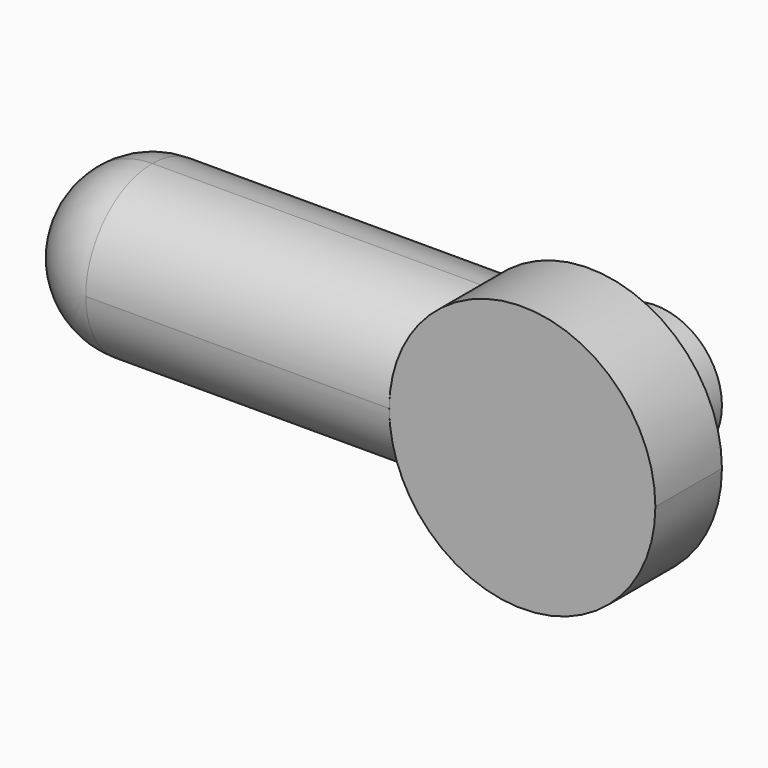
from build123d import *

# Parameters (mm, degrees)
F1_DEPTH = 6.35
F2_R     = 6.3499
F0_R     = 5.08
F3_DEPTH = 6.35
F4_DEPTH = 6.35


# Not quite as in the source:
# - a fillet or chamfer is up to 0.001 mm smaller than in the source, because OpenCascade refuses the exact size


with BuildPart() as f1:
    # F0 (on Front) → F1 (new body, symmetric)
    with BuildSketch(Plane.XZ):
        with BuildLine():
            Line((12.7, 6.35), (-12.7, 6.35))
            Line((-12.7, 6.35), (-12.7, -6.35))
            Line((-12.7, -6.35), (12.7, -6.35))
            ThreePointArc((12.7, -6.35), (10.471147458, 0), (12.7, 6.35))
        make_face()
        with BuildLine():
            Line((-12.7, -6.35), (-12.7, 6.35))
            ThreePointArc((-12.7, 6.35), (-19.05, 0), (-12.7, -6.35))
        make_face()
    extrude(amount=F1_DEPTH, both=True)

    # F2 (radius 6.35 in the source; OpenCascade refuses exactly that, so slightly less here)
    f2_edges = [f1.edges().sort_by_distance(p)[0] for p in [
        (0, -6.35, 6.35),
        (0, 6.35, 6.35),
        (0, -6.35, -6.35),
        (0, 6.35, -6.35),
    ]]
    fillet(f2_edges, radius=F2_R)

    # F0 (on Front) → F3 (join)
    with BuildSketch(Plane.XZ):
        with BuildLine():
            ThreePointArc((30.791147458, 0), (23.9960502669, 9.5866067556), (12.7, 6.35))
            Line((12.7, 6.35), (12.7, -6.35))
            ThreePointArc((12.7, -6.35), (23.9960502669, -9.5866067556), (30.791147458, 0))
        make_face()
        with Locations((20.631147458, 0)):
            Circle(F0_R, mode=Mode.SUBTRACT)
        with BuildLine():
            Line((12.7, -6.35), (12.7, 6.35))
            ThreePointArc((12.7, 6.35), (10.471147458, 0), (12.7, -6.35))
        make_face()
    extrude(amount=F3_DEPTH)

    # F0 (on Front) → F4 (join, symmetric)
    with BuildSketch(Plane.XZ):
        with Locations((20.631147458, 0)):
            Circle(F0_R)
    extrude(amount=F4_DEPTH, both=True)


solid = f1.part
